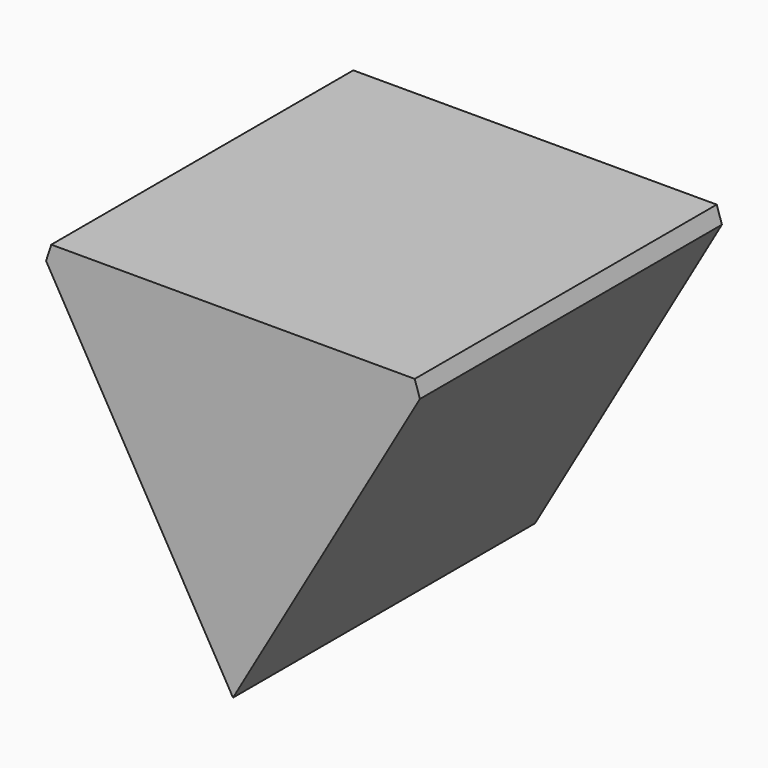
from build123d import *

# Parameters (mm, degrees)
F3_DEPTH = 25


# Not quite as in the source:
# - a feature of the source that left no trace in its solid (it failed there, or was rolled back) is left out
# - the program builds the solid bodies; features that only make, move or delete a surface that nothing else refers to are left out


with BuildPart() as f3:
    # F0 (on Front) → F3 (new body)
    with BuildSketch(Plane.XZ):
        Polygon((12.3791981654, 6.4414001794), (12.0352382333, 7.5), (-12.0352382333, 7.5), (-12.3791981654, 6.4414001794), (0, -15), align=None)
    extrude(amount=F3_DEPTH)


solid = f3.part
